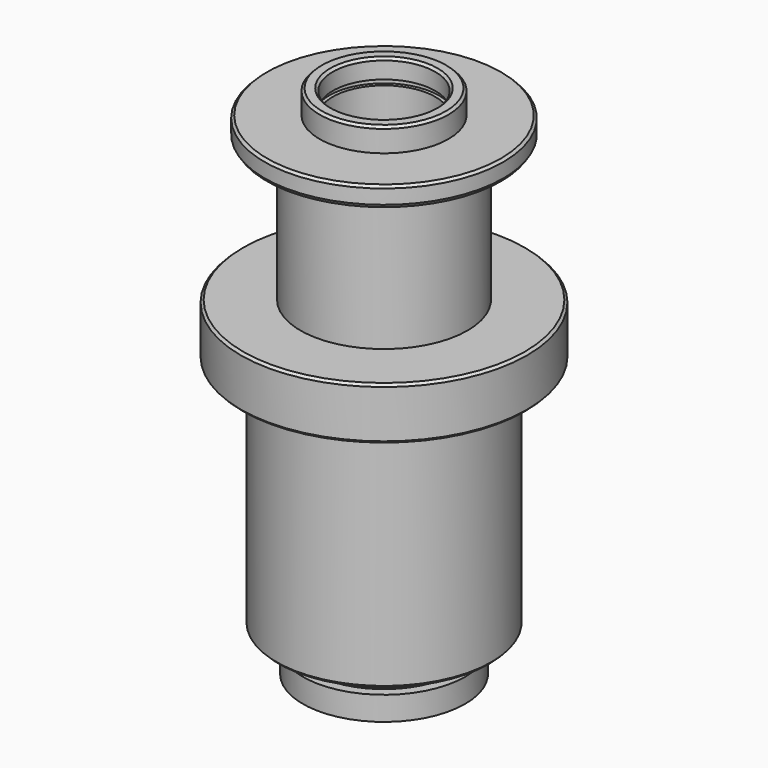
from build123d import *

# Parameters (mm, degrees)
F0_R      = 13.5
F0_R_2    = 10.75
F1_DEPTH  = 5
F2_R      = 25
F2_R_2    = 13.5
F2_R_3    = 10.75
F3_DEPTH  = 7
F4_R      = 17.5
F5_DEPTH  = 27
F6_R      = 30
F6_R_2    = 17.5
F7_DEPTH  = 11
F8_R      = 22.5
F9_DEPTH  = 49
F10_R     = 15
F11_DEPTH = 4
F12_R     = 17
F12_R_2   = 15
F13_DEPTH = 5
F14_R     = 11.5
F15_DEPTH = 37
F16_R     = 10.75
F17_DEPTH = 103.001
F18_SIZE  = 0.5
F19_SIZE2 = 2.99999
F19_SIZE  = 7.49999
F20_SIZE  = 0.5
F22_R     = 11.5
F23_DEPTH = 1.1


# Not quite as in the source:
# - a fillet or chamfer is up to 0.001 mm smaller than in the source, because OpenCascade refuses the exact size


with BuildPart() as f1:
    # F0 (on Top) → F1 (new body)
    with BuildSketch(Plane.XY):
        Circle(F0_R)
        Circle(F0_R_2, mode=Mode.SUBTRACT)
    extrude(amount=F1_DEPTH)

    # F2 (on face) → F3 (join)
    with BuildSketch(Plane(origin=(0, 0, 0), x_dir=(1, 0, 0), z_dir=(0, 0, -1))):
        Circle(F2_R)
        Circle(F2_R_2, mode=Mode.SUBTRACT)
        Circle(F2_R_2)
        Circle(F2_R_3, mode=Mode.SUBTRACT)
    extrude(amount=F3_DEPTH)

    # F4 (on face) → F5 (join)
    with BuildSketch(Plane(origin=(0, 0, -7), x_dir=(1, 0, 0), z_dir=(0, 0, -1))):
        Circle(F4_R)
    extrude(amount=F5_DEPTH)

    # F6 (on face) → F7 (join)
    with BuildSketch(Plane(origin=(0, 0, -34), x_dir=(1, 0, 0), z_dir=(0, 0, -1))):
        Circle(F6_R)
        Circle(F6_R_2, mode=Mode.SUBTRACT)
        Circle(F6_R_2)
    extrude(amount=F7_DEPTH)

    # F8 (on face) → F9 (join)
    with BuildSketch(Plane(origin=(0, 0, -45), x_dir=(1, 0, 0), z_dir=(0, 0, -1))):
        Circle(F8_R)
    extrude(amount=F9_DEPTH)

    # F10 (on face) → F11 (join)
    with BuildSketch(Plane(origin=(0, 0, -94), x_dir=(1, 0, 0), z_dir=(0, 0, -1))):
        Circle(F10_R)
    extrude(amount=F11_DEPTH)

    # F12 (on face) → F13 (join)
    with BuildSketch(Plane(origin=(0, 0, -98), x_dir=(1, 0, 0), z_dir=(0, 0, -1))):
        Circle(F12_R)
        Circle(F12_R_2, mode=Mode.SUBTRACT)
        Circle(F12_R_2)
    extrude(amount=F13_DEPTH)

    # F14 (on face) → F15 (cut)
    with BuildSketch(Plane(origin=(0, 0, -103), x_dir=(1, 0, 0), z_dir=(0, 0, -1))):
        Circle(F14_R)
    extrude(amount=-F15_DEPTH, mode=Mode.SUBTRACT)

    # F16 (on face) → F17 (cut, through all)
    with BuildSketch(Plane.XY):
        Circle(F16_R)
    extrude(amount=-F17_DEPTH, mode=Mode.SUBTRACT)

    # F18
    f18_edges = [f1.edges().sort_by_distance(p)[0] for p in [
        (-11.5, 0, -103),
        (-22.5, 0, -94),
        (-30, 0, -45),
        (-30, 0, -34),
        (-25, 0, 0),
        (-13.5, 0, 5),
        (-10.75, 0, 5),
    ]]
    chamfer(f18_edges, length=F18_SIZE)

    # F19 (size 7.5 and 3 in the source; OpenCascade refuses exactly that, so slightly less here)
    f19_edges = [f1.edges().sort_by_distance(p)[0] for p in [
        (-25, 0, -7),
    ]]
    f19_side = f1.faces().sort_by_distance((-24.292893, 0, -7))[0]
    chamfer(f19_edges, length=F19_SIZE, length2=F19_SIZE2, reference=f19_side)

    # F20
    f20_edges = [f1.edges().sort_by_distance(p)[0] for p in [
        (-25, 0, -4.00001),
    ]]
    chamfer(f20_edges, length=F20_SIZE)

    # F22 (on offset) → F23 (cut)
    with BuildSketch(Plane.XY.offset(1)):
        Circle(F22_R)
    extrude(amount=-F23_DEPTH, mode=Mode.SUBTRACT)


solid = f1.part
